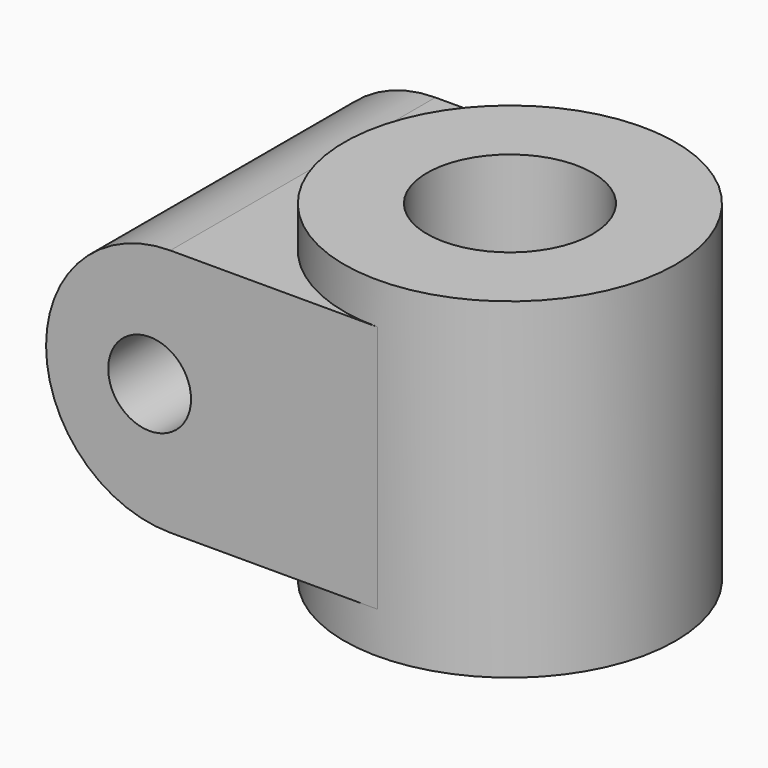
from build123d import *

# Parameters (mm, degrees)
F0_R     = 40
F0_R_2   = 20
F1_DEPTH = 80
F2_W     = 80
F2_H     = 60
F3_DEPTH = 40
F4_R     = 29.99999
F5_DEPTH = 70.001
F6_R     = 10
F7_DEPTH = 80.001


# Not quite as in the source:
# - a fillet or chamfer is up to 0.001 mm smaller than in the source, because OpenCascade refuses the exact size


with BuildPart() as f1:
    # F0 (on Top) → F1 (new body)
    with BuildSketch(Plane.XY):
        Circle(F0_R)
        Circle(F0_R_2, mode=Mode.SUBTRACT)
    extrude(amount=F1_DEPTH)

    # F2 (on Front) → F3 (join, symmetric)
    with BuildSketch(Plane.XZ):
        with Locations((-40, 40)):
            Rectangle(F2_W, F2_H)
    extrude(amount=F3_DEPTH, both=True)

    # F4 (radius 30 in the source; OpenCascade refuses exactly that, so slightly less here)
    f4_edges = [f1.edges().sort_by_distance(p)[0] for p in [
        (-80, 0, 70),
        (-80, 0, 10),
    ]]
    fillet(f4_edges, radius=F4_R)

    # F5 (cut, through all): a face of the model
    f5_faces = [f1.faces().sort_by_distance(p)[0] for p in [
        (-8.4882636316, 0, 70),
    ]]
    extrude(f5_faces, amount=-F5_DEPTH, mode=Mode.SUBTRACT)

    # F6 (on face) → F7 (cut, through all)
    with BuildSketch(Plane.XZ.offset(40)):
        with Locations((-55, 40)):
            Circle(F6_R)
    extrude(amount=-F7_DEPTH, mode=Mode.SUBTRACT)


solid = f1.part
